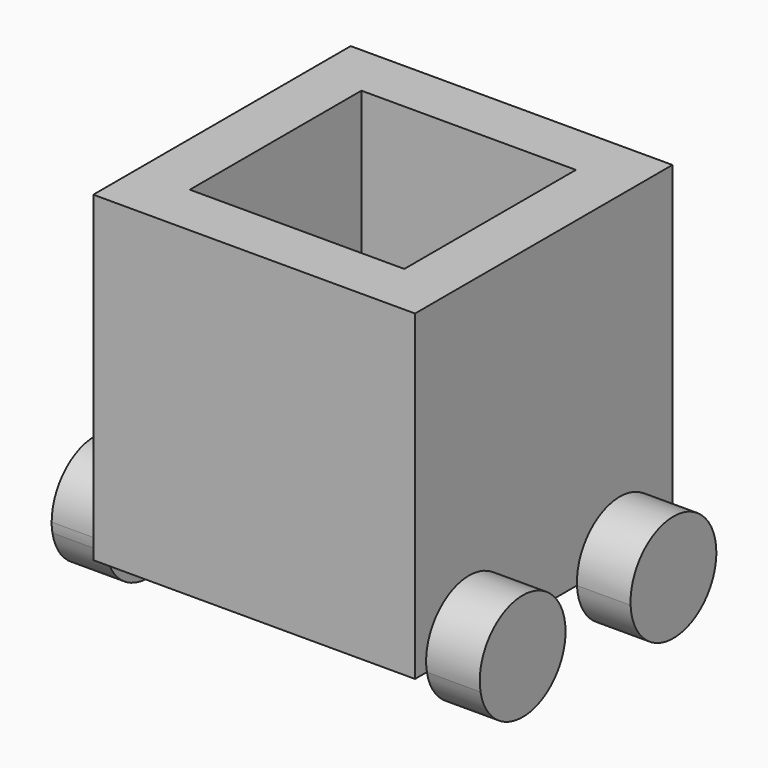
from build123d import *

# Parameters (mm, degrees)
F0_W         = 152.4
F0_H         = 152.4
F1_DEPTH     = 76.2
F4_DEPTH     = 25.4
F5_DEPTH     = 25.4
F8_T         = 25.4
F8_T3_DEPTH  = 101.5109538543
F8_T5_DEPTH  = 100.7130125391
F8_T7_DEPTH  = 100.7009169896
F8_T9_DEPTH  = 101.5275970298
F8_T12_ANGLE = 201.4451187232
F8_T14_ANGLE = 186.7858896324
F8_T16_ANGLE = 201.5912747251
F8_T18_ANGLE = 186.1187901135
F9_R         = 22.86
F10_DEPTH    = 25.4


# Not quite as in the source:
# - a shell that OpenCascade refuses in one call is made with other operations: the cavity is built on its own and cut out
# - the program builds the solid bodies; features that only make, move or delete a surface that nothing else refers to are left out


with BuildPart() as f1:
    # F0 (on Top) → F1 (new body, symmetric)
    with BuildSketch(Plane.XY):
        Rectangle(F0_W, F0_H)
    extrude(amount=F1_DEPTH, both=True)

    # F3 (on face) → F4 (join)
    with BuildSketch(Plane.YZ.offset(76.2)):
        with BuildLine():
            Line((-19.2842212707, -76.2), (-69.1851382603, -76.2))
            ThreePointArc((-69.1851382603, -76.2), (-44.2346797655, -96.8424143834), (-19.2842212707, -76.2))
        make_face()
        with BuildLine():
            ThreePointArc((70.4473548588, -74.8443728776), (44.3692996541, -49.4534248619), (19.6835563439, -76.2))
            Line((19.6835563439, -76.2), (70.4111533737, -76.2))
            ThreePointArc((70.4111533737, -76.2), (70.4383028746, -75.5224280823), (70.4473548588, -74.8443728776))
        make_face()
        with BuildLine():
            ThreePointArc((-19.2842212707, -76.2), (-18.9473148794, -73.8318028232), (-18.8346797655, -71.4424143834))
            ThreePointArc((-18.8346797655, -71.4424143834), (-46.6240682052, -46.1550494973), (-69.1851382603, -76.2))
            Line((-69.1851382603, -76.2), (-19.2842212707, -76.2))
        make_face()
        with BuildLine():
            Line((70.4111533737, -76.2), (19.6835563439, -76.2))
            ThreePointArc((19.6835563439, -76.2), (45.0473548588, -100.2443728776), (70.4111533737, -76.2))
        make_face()
    extrude(amount=F4_DEPTH)

    # F2 (on face) → F5 (join)
    with BuildSketch(Plane(origin=(-76.2, 0, 0), x_dir=(0, -1, 0), z_dir=(-1, 0, 0))):
        with BuildLine():
            ThreePointArc((-19.7216319351, -76.2), (-19.6882420704, -75.4486997337), (-19.6771088623, -74.6967402767))
            ThreePointArc((-19.6771088623, -74.6967402767), (-45.8290683193, -49.3078734849), (-70.4325857895, -76.2))
            Line((-70.4325857895, -76.2), (-19.7216319351, -76.2))
        make_face()
        with BuildLine():
            Line((68.6538224631, -76.2), (18.740809924, -76.2))
            ThreePointArc((18.740809924, -76.2), (43.6973161936, -96.87424135), (68.6538224631, -76.2))
        make_face()
        with BuildLine():
            Line((-19.7216319351, -76.2), (-70.4325857895, -76.2))
            ThreePointArc((-70.4325857895, -76.2), (-45.0771088623, -100.0967402767), (-19.7216319351, -76.2))
        make_face()
        with BuildLine():
            ThreePointArc((69.0973161936, -71.47424135), (41.3240546452, -46.1853578312), (18.740809924, -76.2))
            Line((18.740809924, -76.2), (68.6538224631, -76.2))
            ThreePointArc((68.6538224631, -76.2), (68.9861997123, -73.8475028983), (69.0973161936, -71.47424135))
        make_face()
    extrude(amount=F5_DEPTH)

    # F8: shell of thickness 25.4, made by hand


with BuildPart() as f8_core1:
    # F8_t2: copy of F1
    add(f1.part)

    # the walls: a layer under each face that stays
    f8_faces = [f8_core1.faces().sort_by_distance(p)[0] for p in [
        (0, 76.2, 0),
        (0, 0, -76.2),
        (-76.2, 0, 0),
        (76.2, 0, 0),
        (-76.2, 45.0771088623, -88.1483701384),
        (-76.2, -43.6973161936, -86.537120675),
        (0, -76.2, 0),
        (76.2, -44.2346797655, -86.5212071917),
        (76.2, 45.0473548588, -88.2221864388),
        (-101.6, -43.6973161936, -71.47424135),
        (-101.6, 45.0771088623, -74.6967402767),
        (101.6, -44.2346797655, -71.4424143834),
        (101.6, 45.0473548588, -74.8443728776),
    ]]
    thicken(f8_faces, amount=-F8_T, mode=Mode.SUBTRACT)

    # F8_s4 → F8_t3 (cut)
    with BuildSketch(Plane.XZ.offset(-95.8325857895)):
        Polygon((-75.946, -76.454), (-76.2, -50.8), (-101.6, -50.8), (-101.6, -76.2), align=None)
    extrude(amount=F8_T3_DEPTH, mode=Mode.SUBTRACT)

    # F8_s6 → F8_t5 (cut)
    with BuildSketch(Plane.XZ.offset(-6.659190076)):
        Polygon((-75.946, -76.454), (-76.2, -50.8), (-101.6, -50.8), (-101.6, -76.2), align=None)
    extrude(amount=F8_T5_DEPTH, mode=Mode.SUBTRACT)

    # F8_s8 → F8_t7 (cut)
    with BuildSketch(Plane.XZ.offset(-6.1157787293)):
        Polygon((75.946, -76.454), (76.2, -50.8), (101.6, -50.8), (101.6, -76.2), align=None)
    extrude(amount=F8_T7_DEPTH, mode=Mode.SUBTRACT)

    # F8_s10 → F8_t9 (cut)
    with BuildSketch(Plane.XZ.offset(-95.8111533737)):
        Polygon((75.946, -76.454), (76.2, -50.8), (101.6, -50.8), (101.6, -76.2), align=None)
    extrude(amount=F8_T9_DEPTH, mode=Mode.SUBTRACT)

    # F8_s11 → F8_t12 (revolve, cut)
    with BuildSketch(Plane(origin=(0, 11.5532213455, -61.0120114659), x_dir=(1, 0, 0), z_dir=(0, 0.1860534902, -0.9825396169))):
        Polygon((-76.454, 81.8863763725), (-50.8, 81.6323763725), (-50.8, 56.2323763725), (-76.2, 56.2323763725), align=None)
    revolve(axis=Axis((-76.2, -43.6973161936, -71.47424135), (-1, 0, 0)), revolution_arc=F8_T12_ANGLE, mode=Mode.SUBTRACT)

    # F8_s13 → F8_t14 (revolve, cut)
    with BuildSketch(Plane(origin=(0, 4.5709526713, -77.0982440355), x_dir=(1, 0, 0), z_dir=(0, 0.0591834537, -0.9982471231))):
        Polygon((-76.454, -14.9232831726), (-50.8, -15.1772831726), (-50.8, -40.5772831726), (-76.2, -40.5772831726), align=None)
    revolve(axis=Axis((-76.2, 45.0771088623, -74.6967402767), (-1, 0, 0)), revolution_arc=F8_T14_ANGLE, mode=Mode.SUBTRACT)

    # F8_s15 → F8_t16 (revolve, cut)
    with BuildSketch(Plane(origin=(0, -14.6967131461, -77.0747519679), x_dir=(1, 0, 0), z_dir=(0, -0.1873065203, -0.9823015155))):
        Polygon((76.454, 4.4161629306), (50.8, 4.6701629306), (50.8, 30.0701629306), (76.2, 30.0701629306), align=None)
    revolve(axis=Axis((76.2, -44.2346797655, -71.4424143834), (1, 0, 0)), revolution_arc=F8_T16_ANGLE, mode=Mode.SUBTRACT)

    # F8_s17 → F8_t18 (revolve, cut)
    with BuildSketch(Plane(origin=(0, -3.860520311, -72.2303778943), x_dir=(1, 0, 0), z_dir=(0, -0.0533711465, -0.9985747447))):
        Polygon((76.454, -74.63168087), (50.8, -74.37768087), (50.8, -48.97768087), (76.2, -48.97768087), align=None)
    revolve(axis=Axis((76.2, 45.0473548588, -74.8443728776), (1, 0, 0)), revolution_arc=F8_T18_ANGLE, mode=Mode.SUBTRACT)


with BuildPart() as f1_1:
    add(f1.part)

    # what is left inside the walls is the cavity
    f8_cavity = [f8_core1.part.solids().sort_by_distance(p)[0] for p in [
        (-50.546, 0, -8.466667),
    ]]
    add(f8_cavity, mode=Mode.SUBTRACT)


with BuildPart() as f10:
    # F9 (on face) → F10 (new body)
    with BuildSketch(Plane.XY):
        Circle(F9_R)
    extrude(amount=F10_DEPTH)


solid = Compound([f1_1.part, f10.part])
